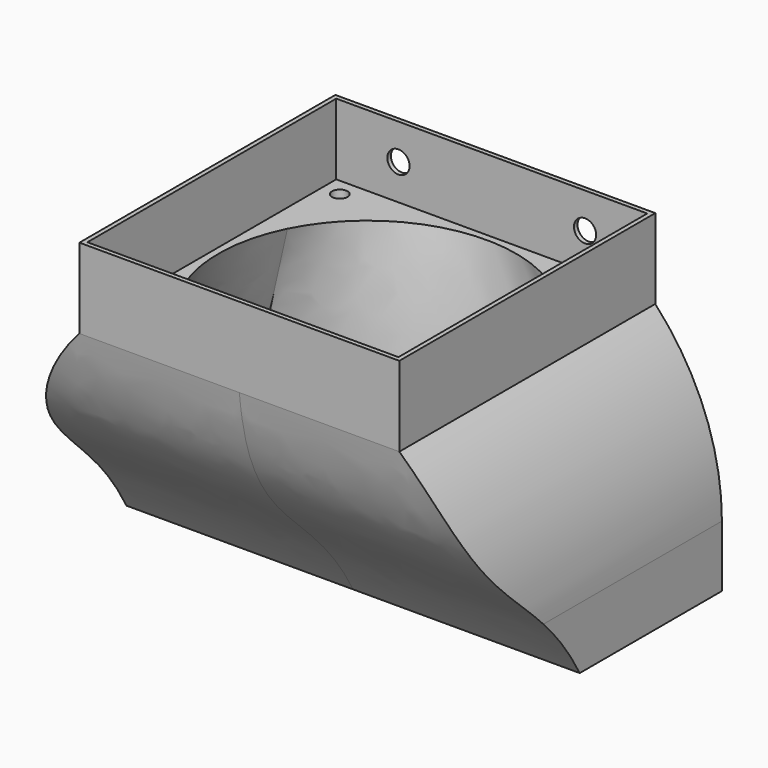
from build123d import *

# Parameters (mm, degrees)
F3_W          = 72
F3_H          = 72
F3_R          = 1.75
F5_DEPTH      = 18
F2_W          = 70
F2_H          = 70
F2_R          = 2
F2_R_2        = 33.5
F7_DEPTH      = 16.001
F8_DEPTH      = 51
F8_DEPTH_BACK = 51
F4_W          = 96
F4_H          = 26
F10_R         = 2.5
F11_DEPTH     = 36.0010001
F12_DEPTH     = 24
F13_T1_DEPTH  = 262.7223112276


# Not quite as in the source:
# - a fillet or chamfer that OpenCascade refuses, or shapes differently, is made with other operations: its cross-section is extruded or revolved along the edge and cut away or added
# - the arcs of a loft's sections are written as splines that run evenly, so that the points pair up as in the source's solid


with BuildPart() as f5:
    # F3 (on Top) → F5 (new body)
    with BuildSketch(Plane.XY):
        Rectangle(F3_W, F3_H)
        with Locations((-31, -31)):
            Circle(F3_R, mode=Mode.SUBTRACT)
        with Locations((31, -31)):
            Circle(F3_R, mode=Mode.SUBTRACT)
        with Locations((-31, 31)):
            Circle(F3_R, mode=Mode.SUBTRACT)
        with Locations((31, 31)):
            Circle(F3_R, mode=Mode.SUBTRACT)
    extrude(amount=-F5_DEPTH)

    # F2 (on offset) → F7 (cut, through all)
    with BuildSketch(Plane.XY.offset(-16)):
        Rectangle(F2_W, F2_H)
        with Locations((-31, -31)):
            Circle(F2_R, mode=Mode.SUBTRACT)
        with Locations((31, -31)):
            Circle(F2_R, mode=Mode.SUBTRACT)
        with Locations((-31, 31)):
            Circle(F2_R, mode=Mode.SUBTRACT)
        Circle(F2_R_2, mode=Mode.SUBTRACT)
        with Locations((31, 31)):
            Circle(F2_R, mode=Mode.SUBTRACT)
        with Locations((-31, 31)):
            Circle(F2_R)
        Circle(F2_R_2)
        with Locations((31, 31)):
            Circle(F2_R)
        with Locations((31, -31)):
            Circle(F2_R)
        with Locations((-31, -31)):
            Circle(F2_R)
    extrude(amount=F7_DEPTH, mode=Mode.SUBTRACT)

    # F6 (on Right) → F8 (join, two sides)
    with BuildSketch(Plane.YZ) as f8_sk:
        with BuildLine():
            add(Edge.make_bspline(
                [(-4, -70), (-16.4795443416, -47.2917743027), (-32.9108946025, -48.374120146), (-36, -18)],
                knots=[0, 0, 0, 0, 61.0573500899, 61.0573500899, 61.0573500899, 61.0573500899], degree=3))
            Line((-4, -70), (26, -70))
            Line((26, -70), (36, -70))
            Line((36, -70), (36, -18))
            Line((36, -18), (-36, -18))
        make_face()
    extrude(amount=F8_DEPTH)
    extrude(f8_sk.sketch, amount=-F8_DEPTH_BACK)

    # F2 (on offset) → F9 section 0
    with BuildSketch(Plane.XY.offset(-16)):
        with BuildLine():
            add(Edge.make_bspline(
                [(-29.9633108985, 14.9816554492), (-30.9438579547, 13.0205613368), (-31.7312346297, 10.9629426487), (-32.8894659049, 6.7335276889), (-33.2602918655, 4.5618359979), (-33.571150125, 0.1877283482), (-33.5111747374, -2.014579452), (-32.9627138727, -6.3652852877), (-32.4742419574, -8.5135757434), (-31.087539012, -12.6736845797), (-30.1893422708, -14.6854000934), (-28.0176874611, -18.4950412808), (-26.7442830911, -20.2928727535), (-23.8711318936, -23.6056439176), (-22.2714561105, -25.1205016941), (-18.8072221146, -27.8090948968), (-16.9427495617, -28.9827638423), (-14.9816554492, -29.9633108985)],
                knots=[0, 0, 0, 0, 0.125, 0.125, 0.25, 0.25, 0.375, 0.375, 0.5, 0.5, 0.625, 0.625, 0.75, 0.75, 0.875, 0.875, 1, 1, 1, 1], degree=3))
            add(Edge.make_bspline(
                [(-14.9816554492, -29.9633108985), (-13.0205613368, -30.9438579547), (-10.9629426487, -31.7312346297), (-6.7335276889, -32.8894659049), (-4.5618359979, -33.2602918655), (-0.1877283482, -33.571150125), (2.014579452, -33.5111747374), (6.3652852877, -32.9627138727), (8.5135757434, -32.4742419574), (12.6736845797, -31.087539012), (14.6854000934, -30.1893422708), (18.4950412808, -28.0176874611), (20.2928727535, -26.7442830911), (23.6056439176, -23.8711318936), (25.1205016941, -22.2714561105), (27.8090948968, -18.8072221146), (28.9827638423, -16.9427495617), (29.9633108985, -14.9816554492)],
                knots=[0, 0, 0, 0, 0.125, 0.125, 0.25, 0.25, 0.375, 0.375, 0.5, 0.5, 0.625, 0.625, 0.75, 0.75, 0.875, 0.875, 1, 1, 1, 1], degree=3))
            add(Edge.make_bspline(
                [(29.9633108985, -14.9816554492), (30.9438579547, -13.0205613368), (31.7312346297, -10.9629426487), (32.8894659049, -6.7335276889), (33.2602918655, -4.5618359979), (33.571150125, -0.1877283482), (33.5111747374, 2.014579452), (32.9627138727, 6.3652852877), (32.4742419574, 8.5135757434), (31.087539012, 12.6736845797), (30.1893422708, 14.6854000934), (28.0176874611, 18.4950412808), (26.7442830911, 20.2928727535), (23.8711318936, 23.6056439176), (22.2714561105, 25.1205016941), (18.8072221146, 27.8090948968), (16.9427495617, 28.9827638423), (14.9816554492, 29.9633108985)],
                knots=[0, 0, 0, 0, 0.125, 0.125, 0.25, 0.25, 0.375, 0.375, 0.5, 0.5, 0.625, 0.625, 0.75, 0.75, 0.875, 0.875, 1, 1, 1, 1], degree=3))
            add(Edge.make_bspline(
                [(14.9816554492, 29.9633108985), (13.0205613368, 30.9438579547), (10.9629426487, 31.7312346297), (6.7335276889, 32.8894659049), (4.5618359979, 33.2602918655), (0.1877283482, 33.571150125), (-2.014579452, 33.5111747374), (-6.3652852877, 32.9627138727), (-8.5135757434, 32.4742419574), (-12.6736845797, 31.087539012), (-14.6854000934, 30.1893422708), (-18.4950412808, 28.0176874611), (-20.2928727535, 26.7442830911), (-23.6056439176, 23.8711318936), (-25.1205016941, 22.2714561105), (-27.8090948968, 18.8072221146), (-28.9827638423, 16.9427495617), (-29.9633108985, 14.9816554492)],
                knots=[0, 0, 0, 0, 0.125, 0.125, 0.25, 0.25, 0.375, 0.375, 0.5, 0.5, 0.625, 0.625, 0.75, 0.75, 0.875, 0.875, 1, 1, 1, 1], degree=3))
        make_face()
    # F4 (on offset) → F9 section 1
    with BuildSketch(Plane.XY.offset(-70)):
        with Locations((0, 11)):
            Rectangle(F4_W, F4_H)
    loft(ruled=True, mode=Mode.SUBTRACT)

    # F10 (on Front) → F11 (cut, through all)
    with BuildSketch(Plane.XZ):
        with Locations((-21, -8)):
            Circle(F10_R)
        with Locations((21, -8)):
            Circle(F10_R)
    extrude(amount=-F11_DEPTH, mode=Mode.SUBTRACT)

    # F3 (on Top) → F12 (cut)
    with BuildSketch(Plane.XY):
        with Locations((-31, 31)):
            Circle(F3_R)
        with Locations((31, 31)):
            Circle(F3_R)
        with Locations((-31, -31)):
            Circle(F3_R)
        with Locations((31, -31)):
            Circle(F3_R)
    extrude(amount=-F12_DEPTH, mode=Mode.SUBTRACT)

    # F13: fillet of radius 56 on 2 edges, made by hand

    # F13_s2 → F13_t1 (cut)
    with BuildSketch(Plane.XZ.offset(-131.3611556138)):
        with BuildLine():
            ThreePointArc((-51, -56.1444622455), (-47.1152568832, -35.6505607136), (-36, -18))
            Line((-36, -18), (-51, -18))
            Line((-51, -18), (-51, -56.1444622455))
        make_face()
        with BuildLine():
            ThreePointArc((51, -56.1444622455), (47.1152568832, -35.6505607136), (36, -18))
            Line((36, -18), (51, -18))
            Line((51, -18), (51, -56.1444622455))
        make_face()
    extrude(amount=F13_T1_DEPTH, mode=Mode.SUBTRACT)


solid = f5.part
